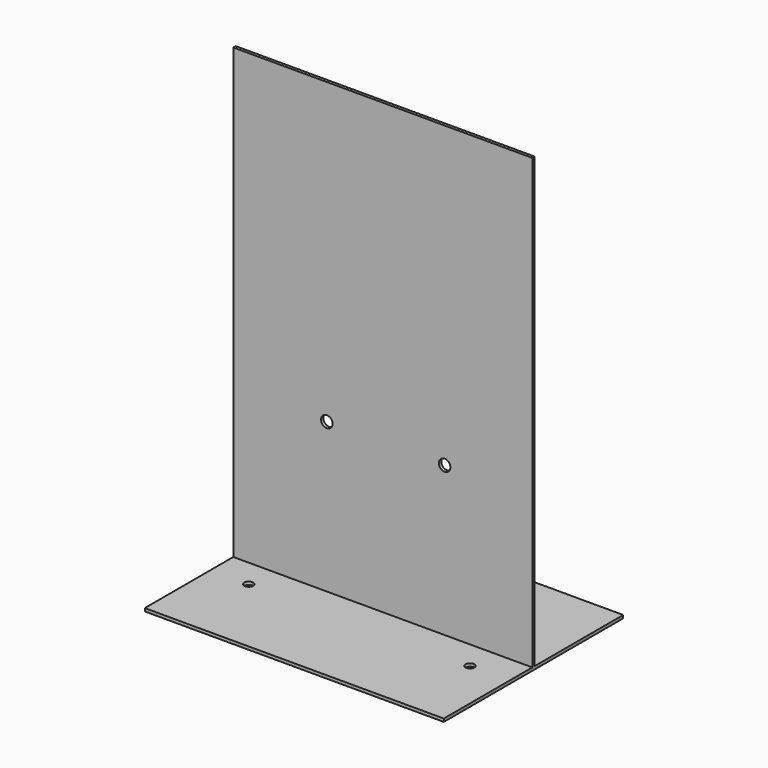
from build123d import *

# Parameters (mm, degrees)
F0_W     = 200
F0_H     = 150
F1_DEPTH = 2
F2_W     = 148
F2_H     = 2
F2_W_2   = 25.5013404053
F3_DEPTH = 300
F5_DEPTH = 2.001
F6_R     = 3.85
F7_DEPTH = 2


with BuildPart() as f1:
    # F0 (on Top) → F1 (new body)
    with BuildSketch(Plane.XY):
        with Locations((0.4986595947, -11.6955466568)):
            Rectangle(F0_W, F0_H)
    extrude(amount=F1_DEPTH)

    # F2 (on face) → F3 (join)
    with BuildSketch(Plane.XY.offset(2)):
        with Locations((0, -11.6955466568)):
            Rectangle(F2_W, F2_H)
        Polygon((100.4986595947, -10.6955466568), (74, -10.6955466568), (74, -12.6955466568), (100.4986595947, -12.6955466568), (100.4986595947, -11.6955466568), align=None)
        with Locations((-86.7506702027, -11.6955466568)):
            Rectangle(F2_W_2, F2_H)
    extrude(amount=F3_DEPTH)

    # F2 (on face) → F5 (cut, through all)
    with BuildSketch(Plane.XY.offset(2)):
        with BuildLine():
            Line((-71, -31.6955466568), (-74, -31.6955466568))
            Line((-74, -31.6955466568), (-74, -34.6955466568))
            ThreePointArc((-74, -34.6955466568), (-71.8786796564, -33.8168670004), (-71, -31.6955466568))
        make_face()
        with BuildLine():
            ThreePointArc((-71, -31.6955466568), (-71.8786796564, -29.5742263133), (-74, -28.6955466568))
            Line((-74, -28.6955466568), (-74, -31.6955466568))
            Line((-74, -31.6955466568), (-71, -31.6955466568))
        make_face()
        with BuildLine():
            ThreePointArc((-74, -28.6955466568), (-76.1213203436, -29.5742263133), (-77, -31.6955466568))
            Line((-77, -31.6955466568), (-74, -31.6955466568))
            Line((-74, -31.6955466568), (-74, -28.6955466568))
        make_face()
        with BuildLine():
            Line((-74, -31.6955466568), (-77, -31.6955466568))
            ThreePointArc((-77, -31.6955466568), (-76.1213203436, -33.8168670004), (-74, -34.6955466568))
            Line((-74, -34.6955466568), (-74, -31.6955466568))
        make_face()
        with BuildLine():
            Line((74, -31.6955466568), (74, -28.6955466568))
            ThreePointArc((74, -28.6955466568), (71.8786796564, -29.5742263133), (71, -31.6955466568))
            Line((71, -31.6955466568), (74, -31.6955466568))
        make_face()
        with BuildLine():
            Line((74, -31.6955466568), (71, -31.6955466568))
            ThreePointArc((71, -31.6955466568), (71.8786796564, -33.8168670004), (74, -34.6955466568))
            Line((74, -34.6955466568), (74, -31.6955466568))
        make_face()
        with BuildLine():
            Line((77, -31.6955466568), (74, -31.6955466568))
            Line((74, -31.6955466568), (74, -34.6955466568))
            ThreePointArc((74, -34.6955466568), (76.1213203436, -33.8168670004), (77, -31.6955466568))
        make_face()
        with BuildLine():
            ThreePointArc((77, -31.6955466568), (76.1213203436, -29.5742263133), (74, -28.6955466568))
            Line((74, -28.6955466568), (74, -31.6955466568))
            Line((74, -31.6955466568), (77, -31.6955466568))
        make_face()
        with BuildLine():
            ThreePointArc((-71, 8.3044533432), (-71.8786796564, 10.4257736867), (-74, 11.3044533432))
            Line((-74, 11.3044533432), (-74, 8.3044533432))
            Line((-74, 8.3044533432), (-71, 8.3044533432))
        make_face()
        with BuildLine():
            Line((-71, 8.3044533432), (-74, 8.3044533432))
            Line((-74, 8.3044533432), (-74, 5.3044533432))
            ThreePointArc((-74, 5.3044533432), (-71.8786796564, 6.1831329996), (-71, 8.3044533432))
        make_face()
        with BuildLine():
            Line((-74, 8.3044533432), (-77, 8.3044533432))
            ThreePointArc((-77, 8.3044533432), (-76.1213203436, 6.1831329996), (-74, 5.3044533432))
            Line((-74, 5.3044533432), (-74, 8.3044533432))
        make_face()
        with BuildLine():
            ThreePointArc((-74, 11.3044533432), (-76.1213203436, 10.4257736867), (-77, 8.3044533432))
            Line((-77, 8.3044533432), (-74, 8.3044533432))
            Line((-74, 8.3044533432), (-74, 11.3044533432))
        make_face()
        with BuildLine():
            Line((77, 8.3044533432), (74, 8.3044533432))
            Line((74, 8.3044533432), (74, 5.3044533432))
            ThreePointArc((74, 5.3044533432), (76.1213203436, 6.1831329996), (77, 8.3044533432))
        make_face()
        with BuildLine():
            ThreePointArc((77, 8.3044533432), (76.1213203436, 10.4257736867), (74, 11.3044533432))
            Line((74, 11.3044533432), (74, 8.3044533432))
            Line((74, 8.3044533432), (77, 8.3044533432))
        make_face()
        with BuildLine():
            Line((74, 8.3044533432), (74, 11.3044533432))
            ThreePointArc((74, 11.3044533432), (71.8786796564, 10.4257736867), (71, 8.3044533432))
            Line((71, 8.3044533432), (74, 8.3044533432))
        make_face()
        with BuildLine():
            Line((74, 5.3044533432), (74, 8.3044533432))
            Line((74, 8.3044533432), (71, 8.3044533432))
            ThreePointArc((71, 8.3044533432), (71.8786796564, 6.1831329996), (74, 5.3044533432))
        make_face()
    extrude(amount=-F5_DEPTH, mode=Mode.SUBTRACT)

    # F6 (on face) → F7 (cut)
    with BuildSketch(Plane(origin=(0, -10.6955466568, 0), x_dir=(-1, 0, 0), z_dir=(0, 1, 0))):
        with Locations((-41.8486595947, 102)):
            Circle(F6_R)
        with Locations((36.9513404053, 102)):
            Circle(F6_R)
    extrude(amount=-F7_DEPTH, mode=Mode.SUBTRACT)


solid = f1.part
